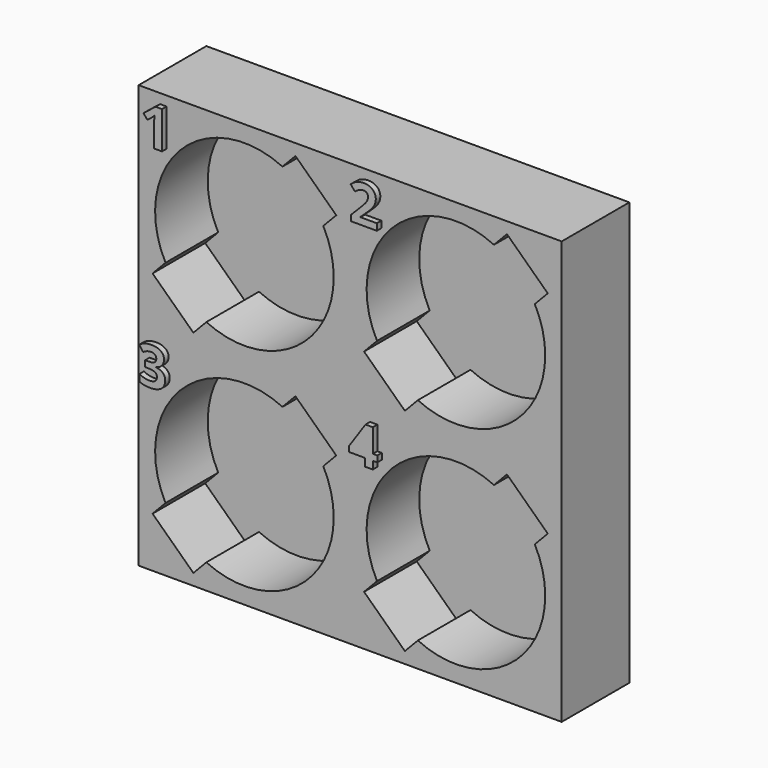
from build123d import *

# Parameters (mm, degrees)
F0_W         = 11.25
F0_H         = 11.25
F1_DEPTH     = 4.5
F3_DEPTH     = 3.5
F8_TEXT_SIZE = 2.7777777778
F9_DEPTH     = 0.3
F10_DEPTH    = 0.3


# Not quite as in the source:
# - Text() gives the source's letters only with a copy of the font that has no kerning and outlines rounded to 1/6400 em; it was checked with that copy


with BuildPart() as f1:
    # F0 (on Front) → F1 (new body)
    with BuildSketch(Plane.XZ):
        Rectangle(F0_W, F0_H)
    extrude(amount=-F1_DEPTH)

    # F2 (on Front) → F3 (cut)
    with BuildSketch(Plane.XZ):
        with BuildLine():
            ThreePointArc((-2.0242524748, -4.2970806274), (2.5443369219, -4.0110908277), (4.75, 0))
            ThreePointArc((4.75, 0), (4.6093152516, 1.147481116), (4.1955945635, 2.2269904038))
            ThreePointArc((4.1955945635, 2.2269904038), (3.277642854, 3.4379583071), (2.0242524748, 4.2970806274))
            ThreePointArc((2.0242524748, 4.2970806274), (-3.4379583071, 3.277642854), (-4.1955945635, -2.2269904038))
            ThreePointArc((-4.1955945635, -2.2269904038), (-3.277642854, -3.4379583071), (-2.0242524748, -4.2970806274))
        make_face()
        with BuildLine():
            ThreePointArc((2.0242524748, 4.2970806274), (3.277642854, 3.4379583071), (4.1955945635, 2.2269904038))
            Line((4.1955945635, 2.2269904038), (4.8856246381, 2.9507711))
            Line((4.8856246381, 2.9507711), (2.7142825494, 5.0208613236))
            Line((2.7142825494, 5.0208613236), (2.0242524748, 4.2970806274))
        make_face()
        with BuildLine():
            Line((-2.7142825494, -5.0208613236), (-2.0242524748, -4.2970806274))
            ThreePointArc((-2.0242524748, -4.2970806274), (-3.277642854, -3.4379583071), (-4.1955945635, -2.2269904038))
            Line((-4.1955945635, -2.2269904038), (-4.8856246381, -2.9507711))
            Line((-4.8856246381, -2.9507711), (-2.7142825494, -5.0208613236))
        make_face()
    extrude(amount=-F3_DEPTH, mode=Mode.SUBTRACT)


with BuildPart() as f4_1:
    # F4: copy of F1
    add(f1.part.moved(Location((-11.25, 0, 0))))


with BuildPart() as f5_1:
    # F5: copy of F1
    add(f1.part.moved(Location((0, 0, 11.25))))


with BuildPart() as f6_1:
    # F6: copy of F1
    add(f1.part.moved(Location((-11.25, 0, 11.25))))


with BuildPart() as f1_1:
    add(f1.part)

    # F7: union F4_1, F5_1, F6_1
    add(f4_1.part)
    add(f5_1.part)
    add(f6_1.part)

    # F8 (on face) → F9 (join)
    with BuildSketch(Plane.XZ):
        with Locations((-16.5388454861, 14.375)):
            Text('1', F8_TEXT_SIZE, font='Open Sans', font_style=FontStyle.BOLD, text_align=(TextAlign.LEFT, TextAlign.BOTTOM))
        with Locations((-5.4637586806, 14.375)):
            Text('2', F8_TEXT_SIZE, font='Open Sans', font_style=FontStyle.BOLD, text_align=(TextAlign.LEFT, TextAlign.BOTTOM))
        with Locations((-16.7042100694, 3.125)):
            Text('3', F8_TEXT_SIZE, font='Open Sans', font_style=FontStyle.BOLD, text_align=(TextAlign.LEFT, TextAlign.BOTTOM))
        with Locations((-5.4861111111, 3.125)):
            Text('4', F8_TEXT_SIZE, font='Open Sans', font_style=FontStyle.BOLD, text_align=(TextAlign.LEFT, TextAlign.BOTTOM))
    extrude(amount=F9_DEPTH)

    # F8 (on face) → F10 (join, through all)
    with BuildSketch(Plane.XZ):
        with BuildLine():
            Line((-5.0698784722, 3.8615451389), (-4.5924479167, 3.8615451389))
            Line((-4.5924479167, 3.8615451389), (-4.5924479167, 4.1979166667))
            add(Edge.make_bspline(
                [(-4.5924479167, 4.1979166667), (-4.5924479167, 4.2821180556), (-4.5855034722, 4.4420572917)],
                knots=[0, 0, 0, 1, 1, 1], degree=2))
            add(Edge.make_bspline(
                [(-4.5855034722, 4.4420572917), (-4.5785590278, 4.6019965278), (-4.5746527778, 4.6280381944)],
                knots=[0, 0, 0, 1, 1, 1], degree=2))
            Line((-4.5746527778, 4.6280381944), (-4.5855034722, 4.6280381944))
            add(Edge.make_bspline(
                [(-4.5855034722, 4.6280381944), (-4.6358506944, 4.5164930556), (-4.7061631944, 4.4110243056)],
                knots=[0, 0, 0, 1, 1, 1], degree=2))
            Line((-4.7061631944, 4.4110243056), (-5.0698784722, 3.8615451389))
        make_face()
    extrude(amount=F10_DEPTH)


solid = f1_1.part
